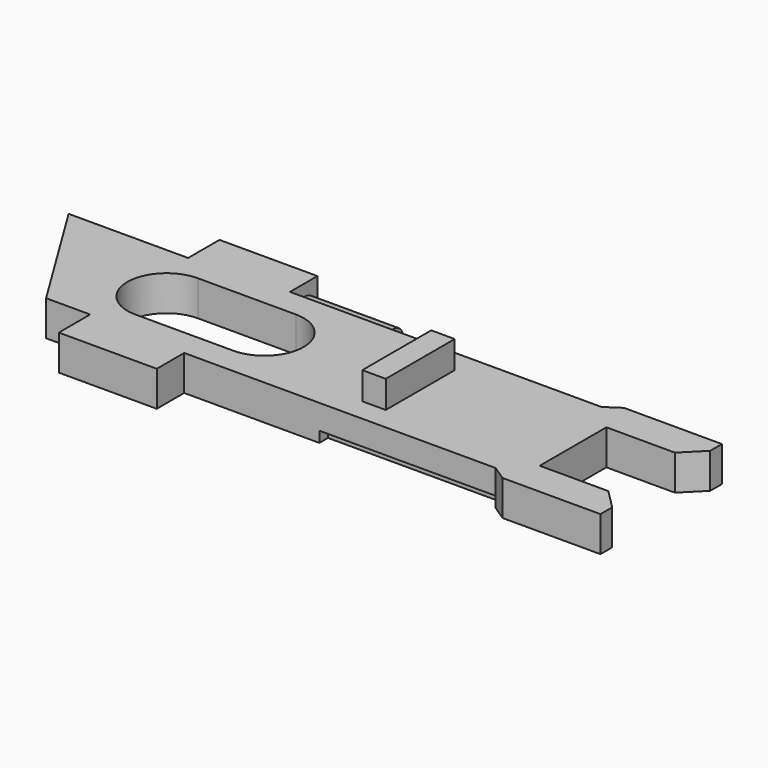
from build123d import *

# Parameters (mm, degrees)
F0_W     = 3.048
F0_H     = 11.176
F1_DEPTH = 4.572
F2_DEPTH = 8.128
F4_DEPTH = 11.43
F5_W     = 22.86
F5_H     = 1.397
F6_DEPTH = 1.397
F7_DEPTH = 1.397


# Not quite as in the source:
# - a feature names something its author has since deleted; it is built from what else it names


with BuildPart() as f1:
    # F0 (on Top) → F1 (new body)
    with BuildSketch(Plane.XY):
        Polygon((18.64257236, -9.8425), (31.34257236, -9.8425), (31.34257236, -7.9375), (28.80257236, -5.3975), (19.91257236, -5.3975), (19.91257236, 5.3975), (28.80257236, 5.3975), (31.34257236, 7.9375), (31.34257236, 9.8425), (18.64257236, 9.8425), (16.73757236, 8.5725), (-23.64842764, 8.5725), (-23.64842764, 13.0175), (-36.34842764, 13.0175), (-36.34842764, 7.9375), (-51.84242764, 7.9375), (-42.06342764, -7.9375), (-36.34842764, -7.9375), (-36.34842764, -13.0175), (-23.64842764, -13.0175), (-23.64842764, -8.5725), (16.73757236, -8.5725), align=None)
        with BuildLine():
            Line((-32.79242764, 5.08), (-20.09242764, 5.08))
            ThreePointArc((-20.09242764, 5.08), (-15.01242764, 0), (-20.09242764, -5.08))
            Line((-20.09242764, -5.08), (-32.79242764, -5.08))
            ThreePointArc((-32.79242764, -5.08), (-37.87242764, 0), (-32.79242764, 5.08))
        make_face(mode=Mode.SUBTRACT)
        with Locations((-1.42342764, 0)):
            Rectangle(F0_W, F0_H, mode=Mode.SUBTRACT)
    extrude(amount=F1_DEPTH)

    # F0 (on Top) → F2 (join)
    with BuildSketch(Plane.XY):
        with Locations((-1.42342764, 0)):
            Rectangle(F0_W, F0_H)
    extrude(amount=F2_DEPTH)

    # F3 (on face) → F4 (join)
    with BuildSketch(Plane.YZ.offset(-23.64842764)):
        with BuildLine():
            ThreePointArc((11.1372406919, 0), (12.1756052203, 0.4675508925), (12.6007169871, 1.524))
            ThreePointArc((12.6007169871, 1.524), (10.0190163668, 2.624139746), (11.0136902567, 0))
            Line((11.0136902567, 0), (11.1372406919, 0))
        make_face()
    extrude(amount=F4_DEPTH)

    # F5 (on face) → F6 (cut)
    with BuildSketch(Plane(origin=(0, 0, 0), x_dir=(1, 0, 0), z_dir=(0, 0, -1))):
        with Locations((5.30757236, 7.874)):
            Rectangle(F5_W, F5_H)
    extrude(amount=-F6_DEPTH, mode=Mode.SUBTRACT)

    # F5 (on face) → F7 (cut)
    with BuildSketch(Plane(origin=(0, 0, 0), x_dir=(1, 0, 0), z_dir=(0, 0, -1))):
        with Locations((5.30757236, -7.874)):
            Rectangle(F5_W, F5_H)
    extrude(amount=-F7_DEPTH, mode=Mode.SUBTRACT)


solid = f1.part
